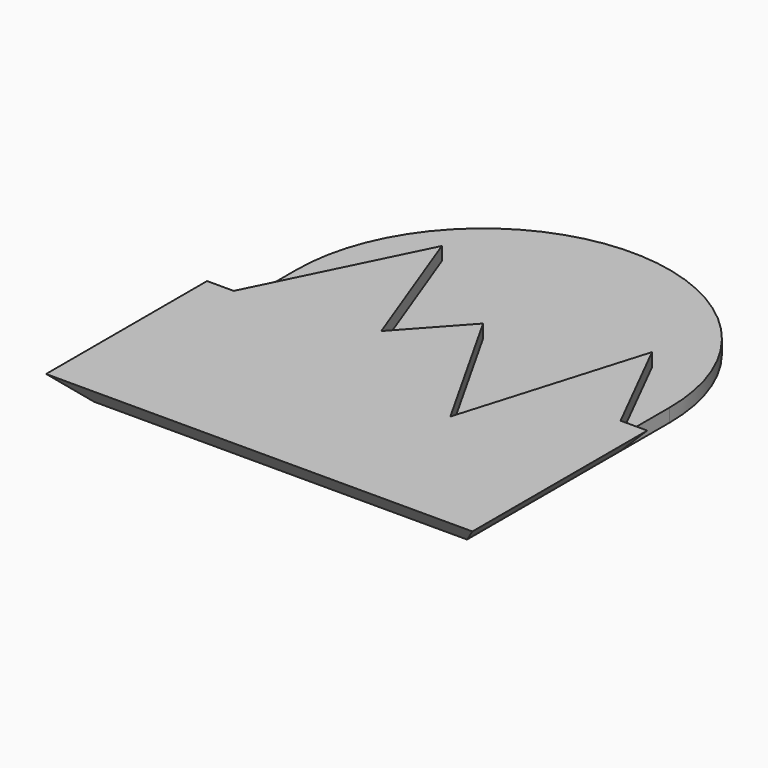
from build123d import *

# Parameters (mm, degrees)
F1_DEPTH = 5
F2_SIZE  = 4.99999
F4_DEPTH = 2.5


# Not quite as in the source:
# - a fillet or chamfer is up to 0.001 mm smaller than in the source, because OpenCascade refuses the exact size


with BuildPart() as f1:
    # F0 (on Top) → F1 (new body)
    with BuildSketch(Plane.XY):
        Polygon((-35, -47.5), (35, -47.5), (35, -11.5), (24.9973740429, 8.3822524399), (14.7012080997, -26.056649141), (0, 0), (-10.1515629949, -11.1895798258), (-20.0927332044, 15.4384202456), (-35, -14.74), align=None)
        Polygon((35, -11.5), (35, -47.5), (-35, -47.5), (-35, -14.74), (-40, -14.74), (-40, -52.5), (40, -52.5), (40, -11.5), align=None)
    extrude(amount=F1_DEPTH)

    # F2 (size 5 in the source; OpenCascade refuses exactly that, so slightly less here)
    f2_edges = [f1.edges().sort_by_distance(p)[0] for p in [
        (40, -32, 0),
        (0, -52.5, 0),
        (-40, -33.62, 0),
    ]]
    chamfer(f2_edges, length=F2_SIZE)

    # F3 (on face) → F4 (join)
    with BuildSketch(Plane(origin=(0, 0, 0), x_dir=(1, 0, 0), z_dir=(0, 0, -1))):
        with BuildLine():
            ThreePointArc((-33.1967424913, 11.0894674339), (-34.5462442763, 5.6175623185), (-35, 0))
            ThreePointArc((-35, 0), (0, -35), (35, 0))
            ThreePointArc((35, 0), (34.6974429309, 4.5921078013), (33.7950026252, 9.1048227638))
            Line((33.7950026252, 9.1048227638), (24.9973740429, -8.3822524399))
            Line((24.9973740429, -8.3822524399), (18.0845360262, 14.74))
            Line((18.0845360262, 14.74), (8.3163343919, 14.74))
            Line((8.3163343919, 14.74), (0, 0))
            Line((0, 0), (-10.1515629949, 11.1895798258))
            Line((-10.1515629949, 11.1895798258), (-20.0927332044, -15.4384202456))
            Line((-20.0927332044, -15.4384202456), (-33.1967424913, 11.0894674339))
        make_face()
        Polygon((14.7012080997, 26.056649141), (8.3163343919, 14.74), (18.0845360262, 14.74), align=None)
        with BuildLine():
            Line((-35, 14.74), (-35, 0))
            ThreePointArc((-35, 0), (-34.5462442763, 5.6175623185), (-33.1967424913, 11.0894674339))
            Line((-33.1967424913, 11.0894674339), (-35, 14.74))
        make_face()
        with BuildLine():
            ThreePointArc((33.7950026252, 9.1048227638), (34.6974429309, 4.5921078013), (35, 0))
            Line((35, 0), (35, 11.5))
            Line((35, 11.5), (33.7950026252, 9.1048227638))
        make_face()
    extrude(amount=-F4_DEPTH)


solid = f1.part
